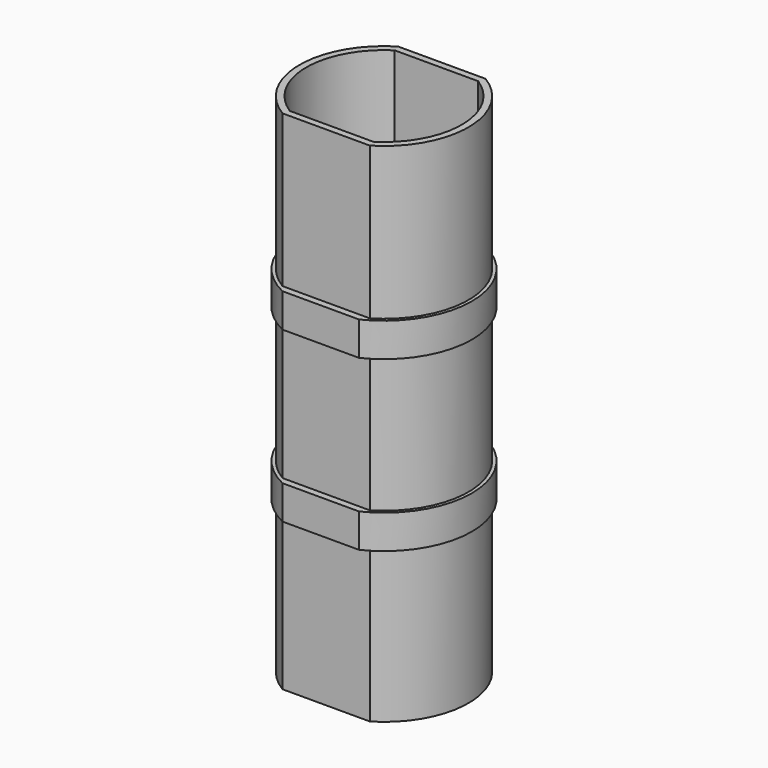
from build123d import *

# Parameters (mm, degrees)
F0_R      = 11.5
F0_R_2    = 6.5
F1_DEPTH  = 75
F2_W      = 40
F2_H      = 22.7775762856
F3_DEPTH  = 75
F5_DEPTH  = 75
F7_DEPTH  = 75
F10_DEPTH = 15
F12_DEPTH = 10


# Not quite as in the source:
# - after a boolean that leaves OpenCascade's solid faulty, fix() repairs it


with BuildPart() as f1:
    # F0 (on Top) → F1 (new body)
    with BuildSketch(Plane.XY):
        Circle(F0_R)
        Circle(F0_R_2, mode=Mode.SUBTRACT)
    extrude(amount=F1_DEPTH)

    # F2 (on face) → F3 (cut, through all)
    with BuildSketch(Plane.XY.offset(75)):
        with Locations((0, -21.0887881428)):
            Rectangle(F2_W, F2_H)
        Polygon((-20, 9.7), (20, 9.7), (20, 33.5304923356), (-20, 28.7892241031), align=None)
    extrude(amount=-F3_DEPTH, mode=Mode.SUBTRACT)

    # F4 (on face) → F5 (join)
    with BuildSketch(Plane.XY.offset(75)):
        with BuildLine():
            Line((6.4621977686, 10.7), (-6.4621977686, 10.7))
            ThreePointArc((-6.4621977686, 10.7), (-12.5, 0), (-6.4621977686, -10.7))
            Line((-6.4621977686, -10.7), (6.4621977686, -10.7))
            ThreePointArc((6.4621977686, -10.7), (12.5, 0), (6.4621977686, 10.7))
        make_face()
        with BuildLine():
            ThreePointArc((-6.1773780846, -9.7), (-11.5, 0), (-6.1773780846, 9.7))
            Line((-6.1773780846, 9.7), (6.1773780846, 9.7))
            ThreePointArc((6.1773780846, 9.7), (11.5, 0), (6.1773780846, -9.7))
            Line((6.1773780846, -9.7), (-6.1773780846, -9.7))
        make_face(mode=Mode.SUBTRACT)
    extrude(amount=-F5_DEPTH)

    # F6 (on face) → F7 (cut)
    with BuildSketch(Plane.XY.offset(75)):
        with BuildLine():
            Line((-6.1773780846, -9.7), (6.1773780846, -9.7))
            ThreePointArc((6.1773780846, -9.7), (11.5, 0), (6.1773780846, 9.7))
            Line((6.1773780846, 9.7), (-6.1773780846, 9.7))
            ThreePointArc((-6.1773780846, 9.7), (-11.5, 0), (-6.1773780846, -9.7))
        make_face()
    extrude(amount=-F7_DEPTH, mode=Mode.SUBTRACT)

    # F9 (on mid) → F10 (join, symmetric)
    with BuildSketch(Plane.XY.offset(37.5)):
        with BuildLine():
            Line((5.6665686266, 11.7), (-5.6665686266, 11.7))
            ThreePointArc((-5.6665686266, 11.7), (-13, 0), (-5.6665686266, -11.7))
            Line((-5.6665686266, -11.7), (5.6665686266, -11.7))
            ThreePointArc((5.6665686266, -11.7), (13, 0), (5.6665686266, 11.7))
        make_face()
        with BuildLine():
            ThreePointArc((-6.1773780846, -9.7), (-11.5, 0), (-6.1773780846, 9.7))
            Line((-6.1773780846, 9.7), (6.1773780846, 9.7))
            ThreePointArc((6.1773780846, 9.7), (11.5, 0), (6.1773780846, -9.7))
            Line((6.1773780846, -9.7), (-6.1773780846, -9.7))
        make_face(mode=Mode.SUBTRACT)
    extrude(amount=F10_DEPTH, both=True)

    add(f1.part.fix(), mode=Mode.REPLACE)

    # F11 (on mid) → F12 (cut, symmetric)
    with BuildSketch(Plane.XY.offset(37.5)):
        with BuildLine():
            Line((-5.6665686266, -11.7), (5.6665686266, -11.7))
            ThreePointArc((5.6665686266, -11.7), (13, 0), (5.6665686266, 11.7))
            Line((5.6665686266, 11.7), (-5.6665686266, 11.7))
            ThreePointArc((-5.6665686266, 11.7), (-13, 0), (-5.6665686266, -11.7))
        make_face()
        with BuildLine():
            ThreePointArc((6.4621977686, 10.7), (12.5, 0), (6.4621977686, -10.7))
            Line((6.4621977686, -10.7), (-6.4621977686, -10.7))
            ThreePointArc((-6.4621977686, -10.7), (-12.5, 0), (-6.4621977686, 10.7))
            Line((-6.4621977686, 10.7), (6.4621977686, 10.7))
        make_face(mode=Mode.SUBTRACT)
    extrude(amount=F12_DEPTH, both=True, mode=Mode.SUBTRACT)

    add(f1.part.fix(), mode=Mode.REPLACE)


solid = f1.part
